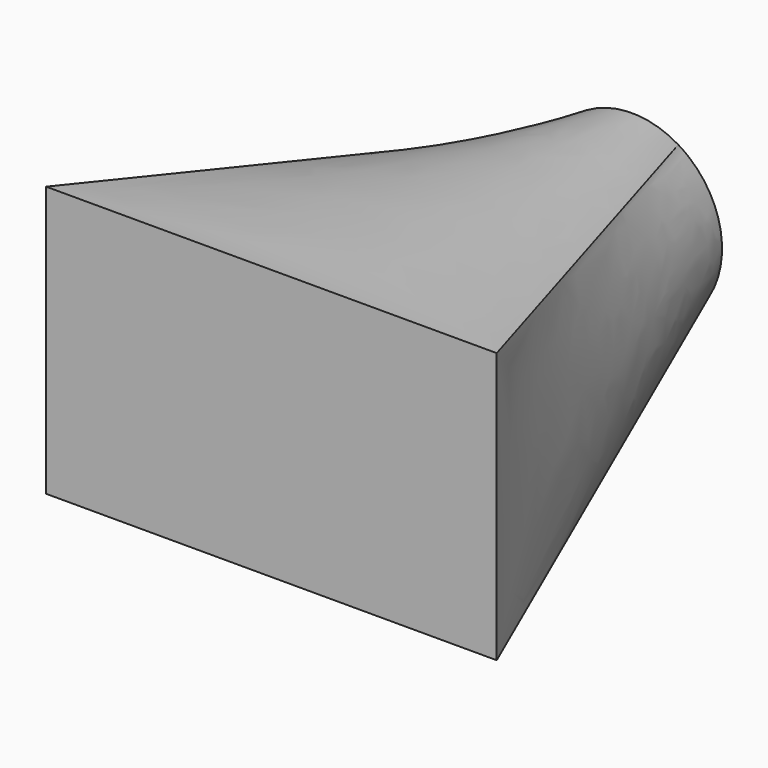
from build123d import *

# Parameters (mm, degrees)
F2_W = 127
F2_H = 76.2


# Not quite as in the source:
# - the arcs of a loft's sections are written as splines that run evenly, so that the points pair up as in the source's solid


with BuildPart() as f3:
    # F2 (on offset) → F3 section 0
    with BuildSketch(Plane.XZ.offset(127)):
        Rectangle(F2_W, F2_H)
    # F0 (on Front) → F3 section 1
    with BuildSketch(Plane.XZ):
        with BuildLine():
            add(Edge.make_bspline(
                [(-21.7803203131, 13.0681921879), (-22.6356314917, 11.6426735568), (-23.3505236623, 10.1329514593), (-24.472067113, 7.0029702123), (-24.8786906608, 5.3827884578), (-25.3680549193, 2.0941466499), (-25.4507835294, 0.4257679146), (-25.2891626016, -2.8951537939), (-25.04481706, -4.5476146508), (-24.2384219474, -7.773195101), (-23.6763923162, -9.3462349355), (-22.2562123309, -12.3525168797), (-21.3980970935, -13.7856846531), (-19.4187089559, -16.457138362), (-18.2974849998, -17.6953582406), (-15.8349554859, -19.9293212464), (-14.4937108189, -20.9250091345), (-13.0681921879, -21.7803203131)],
                knots=[0, 0, 0, 0, 0.125, 0.125, 0.25, 0.25, 0.375, 0.375, 0.5, 0.5, 0.625, 0.625, 0.75, 0.75, 0.875, 0.875, 1, 1, 1, 1], degree=3))
            add(Edge.make_bspline(
                [(-13.0681921879, -21.7803203131), (-11.6426735568, -22.6356314917), (-10.1329514593, -23.3505236623), (-7.0029702123, -24.472067113), (-5.3827884578, -24.8786906608), (-2.0941466499, -25.3680549193), (-0.4257679146, -25.4507835294), (2.8951537939, -25.2891626016), (4.5476146508, -25.04481706), (7.773195101, -24.2384219474), (9.3462349355, -23.6763923162), (12.3525168797, -22.2562123309), (13.7856846531, -21.3980970935), (16.457138362, -19.4187089559), (17.6953582406, -18.2974849998), (19.9293212464, -15.8349554859), (20.9250091345, -14.4937108189), (21.7803203131, -13.0681921879)],
                knots=[0, 0, 0, 0, 0.125, 0.125, 0.25, 0.25, 0.375, 0.375, 0.5, 0.5, 0.625, 0.625, 0.75, 0.75, 0.875, 0.875, 1, 1, 1, 1], degree=3))
            add(Edge.make_bspline(
                [(21.7803203131, -13.0681921879), (22.6356314917, -11.6426735568), (23.3505236623, -10.1329514593), (24.472067113, -7.0029702123), (24.8786906608, -5.3827884578), (25.3680549193, -2.0941466499), (25.4507835294, -0.4257679146), (25.2891626016, 2.8951537939), (25.04481706, 4.5476146508), (24.2384219474, 7.773195101), (23.6763923162, 9.3462349355), (22.2562123309, 12.3525168797), (21.3980970935, 13.7856846531), (19.4187089559, 16.457138362), (18.2974849998, 17.6953582406), (15.8349554859, 19.9293212464), (14.4937108189, 20.9250091345), (13.0681921879, 21.7803203131)],
                knots=[0, 0, 0, 0, 0.125, 0.125, 0.25, 0.25, 0.375, 0.375, 0.5, 0.5, 0.625, 0.625, 0.75, 0.75, 0.875, 0.875, 1, 1, 1, 1], degree=3))
            add(Edge.make_bspline(
                [(13.0681921879, 21.7803203131), (11.6426735568, 22.6356314917), (10.1329514593, 23.3505236623), (7.0029702123, 24.472067113), (5.3827884578, 24.8786906608), (2.0941466499, 25.3680549193), (0.4257679146, 25.4507835294), (-2.8951537939, 25.2891626016), (-4.5476146508, 25.04481706), (-7.773195101, 24.2384219474), (-9.3462349355, 23.6763923162), (-12.3525168797, 22.2562123309), (-13.7856846531, 21.3980970935), (-16.457138362, 19.4187089559), (-17.6953582406, 18.2974849998), (-19.9293212464, 15.8349554859), (-20.9250091345, 14.4937108189), (-21.7803203131, 13.0681921879)],
                knots=[0, 0, 0, 0, 0.125, 0.125, 0.25, 0.25, 0.375, 0.375, 0.5, 0.5, 0.625, 0.625, 0.75, 0.75, 0.875, 0.875, 1, 1, 1, 1], degree=3))
        make_face()
    loft(ruled=True)


solid = f3.part
